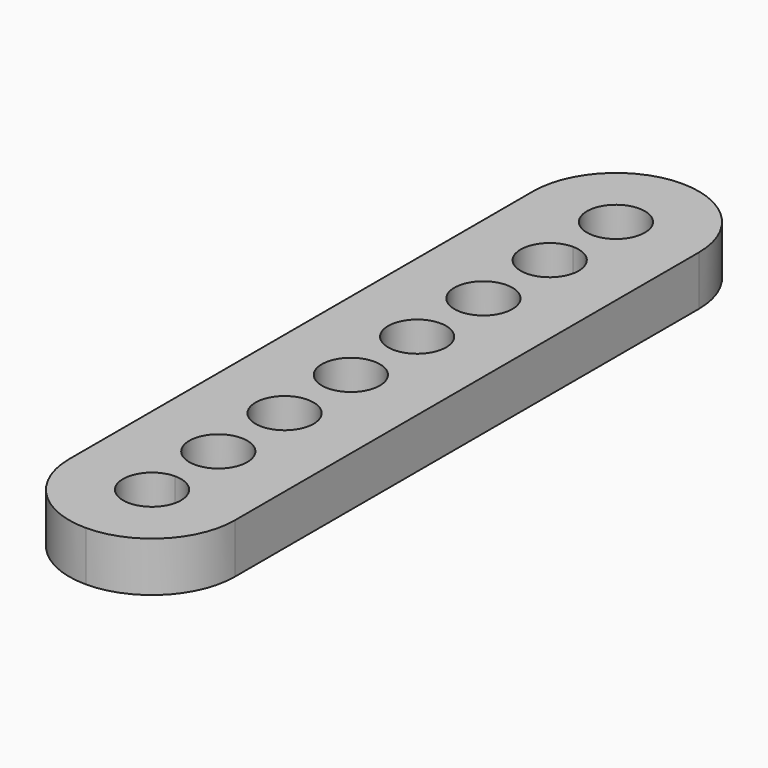
from build123d import *

# Parameters (mm, degrees)
F0_R     = 1.75
F1_DEPTH = 3
F2_R     = 4.99999


# Not quite as in the source:
# - a fillet or chamfer is up to 0.001 mm smaller than in the source, because OpenCascade refuses the exact size


with BuildPart() as f1:
    # F0 (on Top) → F1 (new body)
    with BuildSketch(Plane.XY):
        Polygon((-16.2647291371, -19.261389355), (-16.2647291371, 20.738610645), (-16.2647291371, 25.738610645), (-26.2647291371, 25.738610645), (-26.2647291371, 3.238610645), (-26.2647291371, -19.261389355), (-21.2647291371, -19.261389355), align=None)
        with BuildLine():
            ThreePointArc((-19.5147291371, -14.261389355), (-20.0272922701, -15.4988262221), (-21.2647291371, -16.011389355))
            ThreePointArc((-21.2647291371, -16.011389355), (-23.0147291371, -14.261389355), (-21.2647291371, -12.511389355))
            ThreePointArc((-21.2647291371, -12.511389355), (-20.0272922701, -13.0239524879), (-19.5147291371, -14.261389355))
        make_face(mode=Mode.SUBTRACT)
        with BuildLine():
            ThreePointArc((-19.5147291371, -9.261389355), (-20.0272922701, -10.4988262221), (-21.2647291371, -11.011389355))
            ThreePointArc((-21.2647291371, -11.011389355), (-22.5021660042, -8.0239524879), (-19.5147291371, -9.261389355))
        make_face(mode=Mode.SUBTRACT)
        with Locations((-21.2647291371, -4.261389355)):
            Circle(F0_R, mode=Mode.SUBTRACT)
        with Locations((-21.2647291371, 0.738610645)):
            Circle(F0_R, mode=Mode.SUBTRACT)
        with Locations((-21.2647291371, 5.738610645)):
            Circle(F0_R, mode=Mode.SUBTRACT)
        with Locations((-21.2647291371, 10.738610645)):
            Circle(F0_R, mode=Mode.SUBTRACT)
        with BuildLine():
            ThreePointArc((-19.5147291371, 15.738610645), (-22.5021660042, 14.5011737779), (-21.2647291371, 17.488610645))
            ThreePointArc((-21.2647291371, 17.488610645), (-20.0272922701, 16.9760475121), (-19.5147291371, 15.738610645))
        make_face(mode=Mode.SUBTRACT)
        with BuildLine():
            ThreePointArc((-19.5147291371, 20.738610645), (-20.0272922701, 19.5011737779), (-21.2647291371, 18.988610645))
            ThreePointArc((-21.2647291371, 18.988610645), (-22.5021660042, 21.9760475121), (-19.5147291371, 20.738610645))
        make_face(mode=Mode.SUBTRACT)
    extrude(amount=F1_DEPTH)

    # F2 (radius 5 in the source; OpenCascade refuses exactly that, so slightly less here)
    f2_edges = [f1.edges().sort_by_distance(p)[0] for p in [
        (-16.264729, 25.738611, 1.5),
        (-26.264729, 25.738611, 1.5),
        (-16.264729, -19.261389, 1.5),
        (-26.264729, -19.261389, 1.5),
    ]]
    fillet(f2_edges, radius=F2_R)


solid = f1.part
